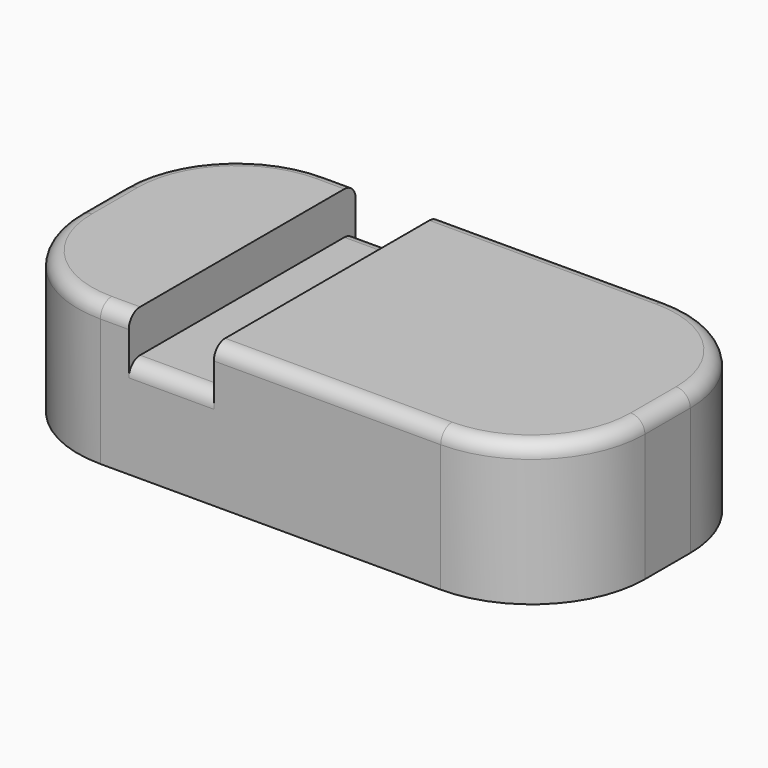
from build123d import *

# Parameters (mm, degrees)
F1_DEPTH = 5
F2_W     = 3
F2_H     = 10
F3_DEPTH = 1.5
F4_R     = 0.5
F6_START = -0.75
F5_R     = 3.3
F6_DEPTH = 3.5


# Not quite as in the source:
# - a feature names something its author has since deleted; it is built from what else it names


with BuildPart() as f1:
    # F0 (on Top) → F1 (new body)
    with BuildSketch(Plane.XY):
        with BuildLine():
            Line((-6, -5), (6, -5))
            ThreePointArc((6, -5), (8.8284271247, -3.8284271247), (10, -1))
            Line((10, -1), (10, 1))
            ThreePointArc((10, 1), (8.8284271247, 3.8284271247), (6, 5))
            Line((6, 5), (-6, 5))
            ThreePointArc((-6, 5), (-8.8284271247, 3.8284271247), (-10, 1))
            Line((-10, 1), (-10, -1))
            ThreePointArc((-10, -1), (-8.8284271247, -3.8284271247), (-6, -5))
        make_face()
    extrude(amount=F1_DEPTH)

    # F2 (on face) → F3 (cut)
    with BuildSketch(Plane.XY.offset(5)):
        with Locations((-3.5, 0)):
            Rectangle(F2_W, F2_H)
    extrude(amount=-F3_DEPTH, mode=Mode.SUBTRACT)

    # F4
    f4_edges = [f1.edges().sort_by_distance(p)[0] for p in [
        (-3.5, -5, 3.5),
        (-3.5, 5, 3.5),
        (2, 5, 5),
        (2, -5, 5),
        (-10, 0, 5),
        (-8.828427, 3.828427, 5),
        (-8.828427, -3.828427, 5),
        (-5.5, 5, 5),
        (-5.5, -5, 5),
        (8.828427, -3.828427, 5),
        (10, 0, 5),
        (8.828427, 3.828427, 5),
    ]]
    fillet(f4_edges, radius=F4_R)

    # F5 (on face) → F6 (cut)
    with BuildSketch(Plane(origin=(0, 0, 0), x_dir=(1, 0, 0), z_dir=(0, 0, -1)).offset(F6_START)):
        with Locations((4.7, 0)):
            Circle(F5_R)
    extrude(amount=-F6_DEPTH, mode=Mode.SUBTRACT)


solid = f1.part
